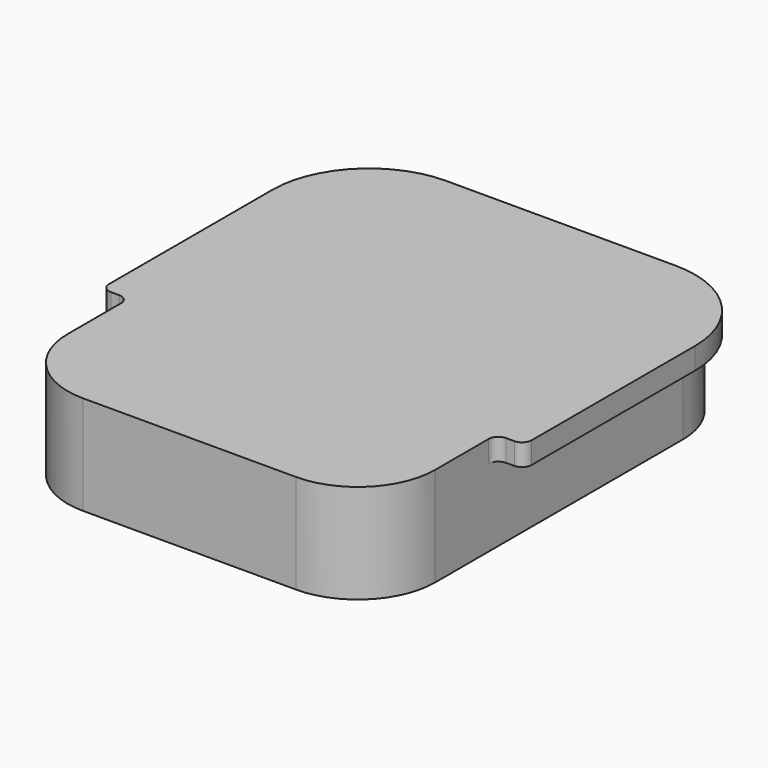
from build123d import *

# Parameters (mm, degrees)
F1_DEPTH     = 10.25
F3_DEPTH     = 2.25
F4_R         = 1
F5_T         = 1.9
F5_T3_DEPTH  = 4.8
F5_T5_DEPTH  = 27.8972844735
F5_T8_ANGLE  = 90.000000001
F5_T10_ANGLE = 90.000000001
F6_R         = 3.75
F6_R_2       = 2.55
F7_DEPTH     = 8
F8_R         = 3.5
F8_R_2       = 1.25
F9_DEPTH     = 8
F10_R        = 3.75
F10_R_2      = 2.55
F11_DEPTH    = 8
F13_DEPTH    = 6


# Not quite as in the source:
# - a shell that OpenCascade refuses in one call is made with other operations: the cavity is built on its own and cut out


with BuildPart() as f1:
    # F0 (on Top) → F1 (new body)
    with BuildSketch(Plane.XY):
        with BuildLine():
            Line((11, 24), (-11, 24))
            ThreePointArc((-11, 24), (-16.6568542495, 21.6568542495), (-19, 16))
            Line((-19, 16), (-19, -16))
            ThreePointArc((-19, -16), (-16.6568542495, -21.6568542495), (-11, -24))
            Line((-11, -24), (11, -24))
            ThreePointArc((11, -24), (16.6568542495, -21.6568542495), (19, -16))
            Line((19, -16), (19, 16))
            ThreePointArc((19, 16), (16.6568542495, 21.6568542495), (11, 24))
        make_face()
    extrude(amount=F1_DEPTH)

    # F2 (on face) → F3 (join)
    with BuildSketch(Plane.XY.offset(10.25)):
        with BuildLine():
            ThreePointArc((-19, 16), (-16.6568542495, 21.6568542495), (-11, 24))
            Line((-11, 24), (-11.85, 24))
            ThreePointArc((-11.85, 24), (-18.9210678119, 21.0710678119), (-21.85, 14))
            Line((-21.85, 14), (-21.85, -8.0972844735))
            Line((-21.85, -8.0972844735), (-19, -8.0972844735))
            Line((-19, -8.0972844735), (-19, 16))
        make_face()
        with BuildLine():
            Line((21.85, -5.7972865179), (21.85, 14))
            ThreePointArc((21.85, 14), (18.9210678119, 21.0710678119), (11.85, 24))
            Line((11.85, 24), (11, 24))
            ThreePointArc((11, 24), (16.6568542495, 21.6568542495), (19, 16))
            Line((19, 16), (19, -8.0972844735))
            Line((19, -8.0972844735), (21.85, -8.0972844735))
            Line((21.85, -8.0972844735), (21.85, -5.7972865179))
        make_face()
    extrude(amount=-F3_DEPTH)

    # F4
    f4_edges = [f1.edges().sort_by_distance(p)[0] for p in [
        (21.85, -8.097284, 9.125),
        (19, -8.097284, 9.125),
        (-21.85, -8.097284, 9.125),
        (-19, -8.097284, 9.125),
    ]]
    fillet(f4_edges, radius=F4_R)

    # F5: shell of thickness 1.9, made by hand


with BuildPart() as f5_core1:
    # F5_t2: copy of F1
    add(f1.part)

    # the walls: a layer under each face that stays
    f5_faces = [f5_core1.faces().sort_by_distance(p)[0] for p in [
        (19, 0, 5.125),
        (0, 0, 10.25),
        (19.2928932188, -8.3901776923, 9.125),
        (16.6568542495, -21.6568542495, 5.125),
        (20.0416666667, -3.5810703946, 8),
        (16.6568542495, 21.6568542495, 4),
        (-21.85, 3.4513577633, 9.125),
        (-18.9210678119, 21.0710678119, 9.125),
        (-20.425, -8.0972844735, 9.125),
        (0, 24, 5.125),
        (-19.2928932188, -8.3901776923, 9.125),
        (18.9210678119, 21.0710678119, 9.125),
        (-19, 0, 5.125),
        (21.85, 3.4513577633, 9.125),
        (-16.6568542495, -21.6568542495, 5.125),
        (0, -24, 5.125),
        (20.425, -8.0972844735, 9.125),
        (-16.6568542495, 21.6568542495, 4),
        (-20.0416666667, -3.5810703946, 8),
    ]]
    thicken(f5_faces, amount=-F5_T, mode=Mode.SUBTRACT)

    # F5_s4 → F5_t3 (cut)
    with BuildSketch(Plane.XZ.offset(6.1972844735)):
        Polygon((19.019, 7.981), (17.1, 8), (17.1, 9.9), (19, 9.9), align=None)
        Polygon((-19.019, 7.981), (-17.1, 8), (-17.1, 9.9), (-19, 9.9), align=None)
    extrude(amount=F5_T3_DEPTH, mode=Mode.SUBTRACT)

    # F5_s6 → F5_t5 (cut)
    with BuildSketch(Plane.XZ.offset(-17.9)):
        Polygon((19.019, 7.981), (17.1, 8), (17.1, 9.9), (19, 9.9), align=None)
        Polygon((-19.019, 7.981), (-17.1, 8), (-17.1, 9.9), (-19, 9.9), align=None)
    extrude(amount=F5_T5_DEPTH, mode=Mode.SUBTRACT)

    # F5_s7 → F5_t8 (revolve, cut)
    with BuildSketch(Plane.YZ.offset(11)):
        Polygon((24.019, 7.981), (24, 9.9), (22.1, 9.9), (22.1, 8), align=None)
    revolve(axis=Axis((11, 16, 8), (0, 0, -1)), revolution_arc=F5_T8_ANGLE, mode=Mode.SUBTRACT)

    # F5_s9 → F5_t10 (revolve, cut)
    with BuildSketch(Plane.XZ.offset(-16)):
        Polygon((-19.019, 7.981), (-17.1, 8), (-17.1, 9.9), (-19, 9.9), align=None)
    revolve(axis=Axis((-11, 16, 8), (0, 0, -1)), revolution_arc=F5_T10_ANGLE, mode=Mode.SUBTRACT)


with BuildPart() as f1_1:
    add(f1.part)

    # what is left inside the walls is the cavity
    f5_cavity = [f5_core1.part.solids().sort_by_distance(p)[0] for p in [
        (0, -7.366667, 0.019),
    ]]
    add(f5_cavity, mode=Mode.SUBTRACT)

    # F6 (on face) → F7 (join)
    with BuildSketch(Plane(origin=(0, 0, 8.35), x_dir=(1, 0, 0), z_dir=(0, 0, -1))):
        with Locations((1.35, 16.1)):
            Circle(F6_R)
        with Locations((1.35, 16.1)):
            Circle(F6_R_2, mode=Mode.SUBTRACT)
    extrude(amount=F7_DEPTH)

    # F8 (on face) → F9 (join)
    with BuildSketch(Plane(origin=(0, 0, 8.35), x_dir=(1, 0, 0), z_dir=(0, 0, -1))):
        with Locations((1.8068233039, 3.7)):
            Circle(F8_R)
        with Locations((1.8068233039, 3.7)):
            Circle(F8_R_2, mode=Mode.SUBTRACT)
    extrude(amount=F9_DEPTH)

    # F10 (on face) → F11 (join)
    with BuildSketch(Plane(origin=(0, 0, 8.35), x_dir=(1, 0, 0), z_dir=(0, 0, -1))):
        with Locations((4.9459114671, -6.65)):
            Circle(F10_R)
        with Locations((4.9459114671, -6.65)):
            Circle(F10_R_2, mode=Mode.SUBTRACT)
    extrude(amount=F11_DEPTH)

    # F12 (on face) → F13 (join)
    with BuildSketch(Plane(origin=(0, 0, 8.35), x_dir=(1, 0, 0), z_dir=(0, 0, -1))):
        with BuildLine():
            ThreePointArc((1.9864868995, 12.4044101382), (1.4880585521, 12.3525422169), (0.987164824, 12.3675945243))
            Line((0.987164824, 12.3675945243), (1.1796292386, 7.1433454088))
            ThreePointArc((1.1796292386, 7.1433454088), (1.6779686553, 7.1976272642), (2.1789513141, 7.1801610227))
            Line((2.1789513141, 7.1801610227), (1.9864868995, 12.4044101382))
        make_face()
    extrude(amount=F13_DEPTH)


solid = f1_1.part
